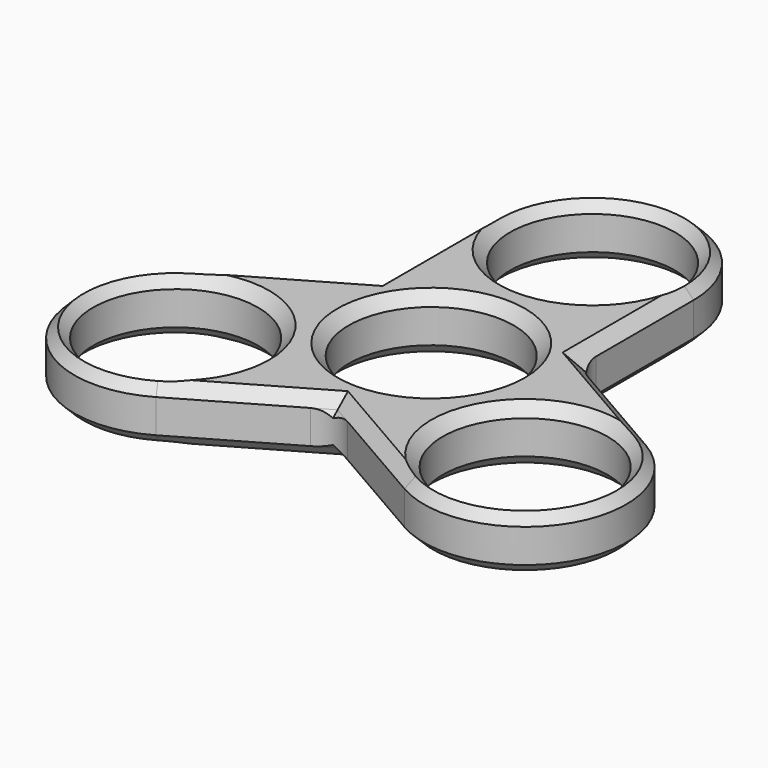
from build123d import *

# Parameters (mm, degrees)
F0_R          = 11.05
F1_DEPTH      = 7.5
F2_T4_DEPTH   = 23.0632958479
F2_T9_DEPTH   = 23.0632958479
F2_T14_DEPTH  = 23.0632958479
F2_T27_DEPTH  = 23.0632958479
F2_T32_DEPTH  = 23.0632958479
F2_T37_DEPTH  = 23.0632958479
F2_T50_DEPTH  = 23.0632958479
F2_T55_DEPTH  = 23.0632958479
F2_T60_DEPTH  = 23.0632958479
F2_T65_DEPTH  = 23.0632958479
F2_T70_DEPTH  = 23.0632958479
F2_T75_DEPTH  = 23.0632958479
F2_T78_ANGLE  = 180
F2_T80_ANGLE  = 180
F2_T82_ANGLE  = 180
F2_T84_ANGLE  = 180
F2_T86_ANGLE  = 180
F2_T88_ANGLE  = 180
F2_T93_DEPTH  = 23.0632958479
F2_T97_DEPTH  = 23.0632958479
F2_T104_DEPTH = 23.0632958479
F2_T108_DEPTH = 23.0632958479
F2_T115_DEPTH = 23.0632958479
F2_T119_DEPTH = 23.0632958479
F2_T126_DEPTH = 23.0632958479
F2_T130_DEPTH = 23.0632958479
F2_T137_DEPTH = 23.0632958479
F2_T141_DEPTH = 23.0632958479
F2_T148_DEPTH = 23.0632958479
F2_T152_DEPTH = 23.0632958479
F3_T4_DEPTH   = 18.9337567297
F3_T10_DEPTH  = 18.9337567297
F3_T16_DEPTH  = 18.9337567297
F3_T22_DEPTH  = 18.9337567297
F3_T28_DEPTH  = 18.9337567297
F3_T34_DEPTH  = 18.9337567297
F3_T40_DEPTH  = 18.9337567297
F3_T46_DEPTH  = 18.9337567297
F3_T52_DEPTH  = 18.9337567297
F3_T58_DEPTH  = 18.9337567297


# Not quite as in the source:
# - a fillet or chamfer that OpenCascade refuses, or shapes differently, is made with other operations: its cross-section is extruded or revolved along the edge and cut away or added


with BuildPart() as f1:
    # F0 (on Top) → F1 (new body)
    with BuildSketch(Plane.XY):
        with BuildLine():
            ThreePointArc((13.55, 27), (0, 40.55), (-13.55, 27))
            Line((-13.55, 27), (-13.55, 7.7942286341))
            Line((-13.55, 7.7942286341), (-30.1826859022, -1.8086570489))
            ThreePointArc((-30.1826859022, -1.8086570489), (-35.1423301235, -20.3183012702), (-16.6326859022, -25.2779454915))
            Line((-16.6326859022, -25.2779454915), (0, -15.6750598085))
            Line((0, -15.6750598085), (16.6326859022, -25.2779454915))
            ThreePointArc((16.6326859022, -25.2779454915), (35.1423301235, -20.3183012702), (30.1826859022, -1.8086570489))
            Line((30.1826859022, -1.8086570489), (13.55, 7.7942286341))
            Line((13.55, 7.7942286341), (13.55, 27))
        make_face()
        with Locations((-23.4076859022, -13.5433012702)):
            Circle(F0_R, mode=Mode.SUBTRACT)
        with Locations((23.4076859022, -13.5433012702)):
            Circle(F0_R, mode=Mode.SUBTRACT)
        Circle(F0_R, mode=Mode.SUBTRACT)
        with Locations((0, 27)):
            Circle(F0_R, mode=Mode.SUBTRACT)
    extrude(amount=F1_DEPTH)

    # F2: chamfer of 1.5 on 20 edges, made by hand


with BuildPart() as f2_tool2:
    # F2_s3 → F2_t4 (new body)
    with BuildSketch(Plane(origin=(-23.4201859022, -13.5216506351, 0), x_dir=(0, 0, 1), z_dir=(0.8660254038, 0.5, 0))):
        Polygon((6, 13.575), (7.5, 12.075), (7.5, 13.575), align=None)
    extrude(amount=F2_T4_DEPTH)

    split(bisect_by=Plane(origin=(-6.7875, -11.7562948564, 0), x_dir=(0, 0, 1), z_dir=(-0.5, -0.8660254038, 0)), keep=Keep.TOP)


with BuildPart() as f1_1:
    add(f1.part)

    # F2_t1: cut F2_tool2
    add(f2_tool2.part, mode=Mode.SUBTRACT)


with BuildPart() as f2_tool7:
    # F2_s8 → F2_t9 (new body)
    with BuildSketch(Plane.XZ.offset(-27)):
        Polygon((-13.55, 6), (-12.05, 7.5), (-13.55, 7.5), align=None)
    extrude(amount=F2_T9_DEPTH)

    split(bisect_by=Plane(origin=(-6.7625, 11.7129935862, 0), x_dir=(0, 0, 1), z_dir=(-0.5, 0.8660254038, 0)), keep=Keep.TOP)


with BuildPart() as f1_2:
    add(f1_1.part)

    # F2_t6: cut F2_tool7
    add(f2_tool7.part, mode=Mode.SUBTRACT)


with BuildPart() as f2_tool12:
    # F2_s13 → F2_t14 (new body)
    with BuildSketch(Plane(origin=(3.4467858029, -1.9900027112, 0), x_dir=(0, 0, 1), z_dir=(0.8660254038, -0.5, 0))):
        Polygon((6, 13.575), (7.5, 12.075), (7.5, 13.575), align=None)
    extrude(amount=F2_T14_DEPTH)

    split(bisect_by=Plane(origin=(6.7875, -11.7562948564, 0), x_dir=(0, 0, 1), z_dir=(0.5, -0.8660254038, 0)), keep=Keep.TOP)


with BuildPart() as f1_3:
    add(f1_2.part)

    # F2_t11: cut F2_tool12
    add(f2_tool12.part, mode=Mode.SUBTRACT)

    # F2_s16 → F2_t17 (revolve, cut)
    with BuildSketch(Plane.XZ.offset(13.5433012702)):
        Polygon((-12.3576859022, 6), (-10.8576859022, 7.5), (-12.3576859022, 7.5), align=None)
    revolve(axis=Axis((-23.4076859022, -13.5433012702, 7.5), (0, 0, 1)), mode=Mode.SUBTRACT)

    # F2_s18 → F2_t19 (revolve, cut)
    with BuildSketch(Plane.XZ):
        Polygon((11.05, 6), (12.55, 7.5), (11.05, 7.5), align=None)
    revolve(axis=Axis((0, 0, 7.5), (0, 0, 1)), mode=Mode.SUBTRACT)

    # F2_s20 → F2_t21 (revolve, cut)
    with BuildSketch(Plane.XZ.offset(-27)):
        Polygon((11.05, 6), (12.55, 7.5), (11.05, 7.5), align=None)
    revolve(axis=Axis((0, 27, 7.5), (0, 0, 1)), mode=Mode.SUBTRACT)

    # F2_s22 → F2_t23 (revolve, cut)
    with BuildSketch(Plane.XZ.offset(13.5433012702)):
        Polygon((34.4576859022, 6), (35.9576859022, 7.5), (34.4576859022, 7.5), align=None)
    revolve(axis=Axis((23.4076859022, -13.5433012702, 7.5), (0, 0, 1)), mode=Mode.SUBTRACT)


with BuildPart() as f2_tool25:
    # F2_s26 → F2_t27 (new body)
    with BuildSketch(Plane.XZ.offset(-27)):
        Polygon((-13.55, 1.5), (-12.05, 0), (-13.55, 0), align=None)
    extrude(amount=F2_T27_DEPTH)

    split(bisect_by=Plane(origin=(-6.7625, 11.7129935862, 0), x_dir=(0, 0, 1), z_dir=(-0.5, 0.8660254038, 0)), keep=Keep.TOP)


with BuildPart() as f1_4:
    add(f1_3.part)

    # F2_t24: cut F2_tool25
    add(f2_tool25.part, mode=Mode.SUBTRACT)


with BuildPart() as f2_tool30:
    # F2_s31 → F2_t32 (new body)
    with BuildSketch(Plane(origin=(-3.4467858029, -1.9900027112, 0), x_dir=(0, 0, 1), z_dir=(-0.8660254038, -0.5, 0))):
        Polygon((1.5, 13.525), (0, 12.025), (0, 13.525), align=None)
    extrude(amount=F2_T32_DEPTH)

    split(bisect_by=Plane.YZ.offset(-13.55), keep=Keep.BOTTOM)


with BuildPart() as f1_5:
    add(f1_4.part)

    # F2_t29: cut F2_tool30
    add(f2_tool30.part, mode=Mode.SUBTRACT)


with BuildPart() as f2_tool35:
    # F2_s36 → F2_t37 (new body)
    with BuildSketch(Plane(origin=(3.4467858029, -1.9900027112, 0), x_dir=(0, 0, 1), z_dir=(0.8660254038, -0.5, 0))):
        Polygon((1.5, 13.575), (0, 12.075), (0, 13.575), align=None)
    extrude(amount=F2_T37_DEPTH)

    split(bisect_by=Plane(origin=(6.7875, -11.7562948564, 0), x_dir=(0, 0, 1), z_dir=(0.5, -0.8660254038, 0)), keep=Keep.TOP)


with BuildPart() as f1_6:
    add(f1_5.part)

    # F2_t34: cut F2_tool35
    add(f2_tool35.part, mode=Mode.SUBTRACT)

    # F2_s39 → F2_t40 (revolve, cut)
    with BuildSketch(Plane.XZ.offset(13.5433012702)):
        Polygon((34.4576859022, 1.5), (35.9576859022, 0), (34.4576859022, 0), align=None)
    revolve(axis=Axis((23.4076859022, -13.5433012702, 0), (0, 0, 1)), mode=Mode.SUBTRACT)

    # F2_s41 → F2_t42 (revolve, cut)
    with BuildSketch(Plane.XZ):
        Polygon((11.05, 1.5), (12.55, 0), (11.05, 0), align=None)
    revolve(axis=Axis((0, 0, 0), (0, 0, 1)), mode=Mode.SUBTRACT)

    # F2_s43 → F2_t44 (revolve, cut)
    with BuildSketch(Plane.XZ.offset(13.5433012702)):
        Polygon((-12.3576859022, 1.5), (-10.8576859022, 0), (-12.3576859022, 0), align=None)
    revolve(axis=Axis((-23.4076859022, -13.5433012702, 0), (0, 0, 1)), mode=Mode.SUBTRACT)

    # F2_s45 → F2_t46 (revolve, cut)
    with BuildSketch(Plane.XZ.offset(-27)):
        Polygon((11.05, 1.5), (12.55, 0), (11.05, 0), align=None)
    revolve(axis=Axis((0, 27, 0), (0, 0, 1)), mode=Mode.SUBTRACT)


with BuildPart() as f2_tool48:
    # F2_s49 → F2_t50 (new body)
    with BuildSketch(Plane(origin=(-23.4201859022, -13.5216506351, 0), x_dir=(0, 0, 1), z_dir=(0.8660254038, 0.5, 0))):
        Polygon((1.5, 13.575), (0, 12.075), (0, 13.575), align=None)
    extrude(amount=F2_T50_DEPTH)

    split(bisect_by=Plane(origin=(-6.7875, -11.7562948564, 0), x_dir=(0, 0, 1), z_dir=(-0.5, -0.8660254038, 0)), keep=Keep.TOP)


with BuildPart() as f1_7:
    add(f1_6.part)

    # F2_t47: cut F2_tool48
    add(f2_tool48.part, mode=Mode.SUBTRACT)


with BuildPart() as f2_tool53:
    # F2_s54 → F2_t55 (new body)
    with BuildSketch(Plane(origin=(23.4201859022, -13.5216506351, 0), x_dir=(0, 0, 1), z_dir=(-0.8660254038, 0.5, 0))):
        Polygon((1.5, 13.525), (0, 12.025), (0, 13.525), align=None)
    extrude(amount=F2_T55_DEPTH)

    split(bisect_by=Plane.YZ.offset(13.55), keep=Keep.TOP)


with BuildPart() as f1_8:
    add(f1_7.part)

    # F2_t52: cut F2_tool53
    add(f2_tool53.part, mode=Mode.SUBTRACT)


with BuildPart() as f2_tool58:
    # F2_s59 → F2_t60 (new body)
    with BuildSketch(Plane(origin=(23.4201859022, -13.5216506351, 0), x_dir=(0, 0, 1), z_dir=(-0.8660254038, 0.5, 0))):
        Polygon((6, 13.525), (7.5, 12.025), (7.5, 13.525), align=None)
    extrude(amount=F2_T60_DEPTH)

    split(bisect_by=Plane.YZ.offset(13.55), keep=Keep.TOP)


with BuildPart() as f1_9:
    add(f1_8.part)

    # F2_t57: cut F2_tool58
    add(f2_tool58.part, mode=Mode.SUBTRACT)


with BuildPart() as f2_tool63:
    # F2_s64 → F2_t65 (new body)
    with BuildSketch(Plane.XZ.offset(-3.9367041521)):
        Polygon((13.55, 1.5), (12.05, 0), (13.55, 0), align=None)
    extrude(amount=-F2_T65_DEPTH)

    split(bisect_by=Plane(origin=(6.7625, 11.7129935862, 0), x_dir=(0, 0, 1), z_dir=(0.5, 0.8660254038, 0)), keep=Keep.TOP)


with BuildPart() as f1_10:
    add(f1_9.part)

    # F2_t62: cut F2_tool63
    add(f2_tool63.part, mode=Mode.SUBTRACT)


with BuildPart() as f2_tool68:
    # F2_s69 → F2_t70 (new body)
    with BuildSketch(Plane.XZ.offset(-3.9367041521)):
        Polygon((13.55, 6), (12.05, 7.5), (13.55, 7.5), align=None)
    extrude(amount=-F2_T70_DEPTH)

    split(bisect_by=Plane(origin=(6.7625, 11.7129935862, 0), x_dir=(0, 0, 1), z_dir=(0.5, 0.8660254038, 0)), keep=Keep.TOP)


with BuildPart() as f1_11:
    add(f1_10.part)

    # F2_t67: cut F2_tool68
    add(f2_tool68.part, mode=Mode.SUBTRACT)


with BuildPart() as f2_tool73:
    # F2_s74 → F2_t75 (new body)
    with BuildSketch(Plane(origin=(-3.4467858029, -1.9900027112, 0), x_dir=(0, 0, 1), z_dir=(-0.8660254038, -0.5, 0))):
        Polygon((6, 13.525), (7.5, 12.025), (7.5, 13.525), align=None)
    extrude(amount=F2_T75_DEPTH)

    split(bisect_by=Plane.YZ.offset(-13.55), keep=Keep.BOTTOM)


with BuildPart() as f1_12:
    add(f1_11.part)

    # F2_t72: cut F2_tool73
    add(f2_tool73.part, mode=Mode.SUBTRACT)

    # F2_s77 → F2_t78 (revolve, cut)
    with BuildSketch(Plane(origin=(-23.4201859022, -13.5216506351, 0), x_dir=(0, 0, 1), z_dir=(0.8660254038, 0.5, 0))):
        Polygon((6, -13.525), (7.5, -12.025), (7.5, -13.525), align=None)
    revolve(axis=Axis((-23.4076859022, -13.5433012702, 7.5), (0, 0, 1)), revolution_arc=F2_T78_ANGLE, mode=Mode.SUBTRACT)

    # F2_s79 → F2_t80 (revolve, cut)
    with BuildSketch(Plane.XZ.offset(-27)):
        Polygon((13.55, 6), (12.05, 7.5), (13.55, 7.5), align=None)
    revolve(axis=Axis((0, 27, 7.5), (0, 0, 1)), revolution_arc=F2_T80_ANGLE, mode=Mode.SUBTRACT)

    # F2_s81 → F2_t82 (revolve, cut)
    with BuildSketch(Plane.XZ.offset(-27)):
        Polygon((13.55, 1.5), (12.05, 0), (13.55, 0), align=None)
    revolve(axis=Axis((0, 27, 0), (0, 0, 1)), revolution_arc=F2_T82_ANGLE, mode=Mode.SUBTRACT)

    # F2_s83 → F2_t84 (revolve, cut)
    with BuildSketch(Plane(origin=(23.4201859022, -13.5216506351, 0), x_dir=(0, 0, 1), z_dir=(-0.8660254038, 0.5, 0))):
        Polygon((6, -13.575), (7.5, -12.075), (7.5, -13.575), align=None)
    revolve(axis=Axis((23.4076859022, -13.5433012702, 7.5), (0, 0, 1)), revolution_arc=F2_T84_ANGLE, mode=Mode.SUBTRACT)

    # F2_s85 → F2_t86 (revolve, cut)
    with BuildSketch(Plane(origin=(23.4201859022, -13.5216506351, 0), x_dir=(0, 0, 1), z_dir=(-0.8660254038, 0.5, 0))):
        Polygon((1.5, -13.575), (0, -12.075), (0, -13.575), align=None)
    revolve(axis=Axis((23.4076859022, -13.5433012702, 0), (0, 0, 1)), revolution_arc=F2_T86_ANGLE, mode=Mode.SUBTRACT)

    # F2_s87 → F2_t88 (revolve, cut)
    with BuildSketch(Plane(origin=(-23.4201859022, -13.5216506351, 0), x_dir=(0, 0, 1), z_dir=(0.8660254038, 0.5, 0))):
        Polygon((1.5, -13.525), (0, -12.025), (0, -13.525), align=None)
    revolve(axis=Axis((-23.4076859022, -13.5433012702, 0), (0, 0, 1)), revolution_arc=F2_T88_ANGLE, mode=Mode.SUBTRACT)


with BuildPart() as f2_tool91:
    # F2_s92 → F2_t93 (new body)
    with BuildSketch(Plane(origin=(-23.4201859022, -13.5216506351, 0), x_dir=(0, 0, 1), z_dir=(0.8660254038, 0.5, 0))):
        Polygon((6, 13.575), (7.5, 12.075), (7.5, 13.575), align=None)
    extrude(amount=F2_T93_DEPTH)

    split(bisect_by=Plane(origin=(-6.7875, -11.7562948564, 0), x_dir=(0, 0, 1), z_dir=(0.5, 0.8660254038, 0)), keep=Keep.TOP)


with BuildPart() as f2_tool95:
    # F2_s96 → F2_t97 (new body)
    with BuildSketch(Plane(origin=(3.4467858029, -1.9900027112, 0), x_dir=(0, 0, 1), z_dir=(0.8660254038, -0.5, 0))):
        Polygon((6, 13.575), (7.5, 12.075), (7.5, 13.575), align=None)
    extrude(amount=F2_T97_DEPTH)

    split(bisect_by=Plane(origin=(6.7875, -11.7562948564, 0), x_dir=(0, 0, 1), z_dir=(-0.5, 0.8660254038, 0)), keep=Keep.TOP)


with BuildPart() as f2_tool91_1:
    add(f2_tool91.part)

    # F2_t99: intersect F2_tool95
    add(f2_tool95.part, mode=Mode.INTERSECT)


with BuildPart() as f1_13:
    add(f1_12.part)

    # F2_t89: cut F2_tool91
    add(f2_tool91_1.part, mode=Mode.SUBTRACT)


with BuildPart() as f2_tool102:
    # F2_s103 → F2_t104 (new body)
    with BuildSketch(Plane.XZ.offset(-27)):
        Polygon((-13.55, 6), (-12.05, 7.5), (-13.55, 7.5), align=None)
    extrude(amount=F2_T104_DEPTH)

    split(bisect_by=Plane(origin=(-6.7625, 11.7129935862, 0), x_dir=(0, 0, 1), z_dir=(0.5, -0.8660254038, 0)), keep=Keep.TOP)


with BuildPart() as f2_tool106:
    # F2_s107 → F2_t108 (new body)
    with BuildSketch(Plane(origin=(-3.4467858029, -1.9900027112, 0), x_dir=(0, 0, 1), z_dir=(-0.8660254038, -0.5, 0))):
        Polygon((6, 13.525), (7.5, 12.025), (7.5, 13.525), align=None)
    extrude(amount=F2_T108_DEPTH)

    split(bisect_by=Plane.YZ.offset(-13.55), keep=Keep.TOP)


with BuildPart() as f2_tool102_1:
    add(f2_tool102.part)

    # F2_t110: intersect F2_tool106
    add(f2_tool106.part, mode=Mode.INTERSECT)


with BuildPart() as f1_14:
    add(f1_13.part)

    # F2_t100: cut F2_tool102
    add(f2_tool102_1.part, mode=Mode.SUBTRACT)


with BuildPart() as f2_tool113:
    # F2_s114 → F2_t115 (new body)
    with BuildSketch(Plane.XZ.offset(-27)):
        Polygon((-13.55, 1.5), (-12.05, 0), (-13.55, 0), align=None)
    extrude(amount=F2_T115_DEPTH)

    split(bisect_by=Plane(origin=(-6.7625, 11.7129935862, 0), x_dir=(0, 0, 1), z_dir=(0.5, -0.8660254038, 0)), keep=Keep.TOP)


with BuildPart() as f2_tool117:
    # F2_s118 → F2_t119 (new body)
    with BuildSketch(Plane(origin=(-3.4467858029, -1.9900027112, 0), x_dir=(0, 0, 1), z_dir=(-0.8660254038, -0.5, 0))):
        Polygon((1.5, 13.525), (0, 12.025), (0, 13.525), align=None)
    extrude(amount=F2_T119_DEPTH)

    split(bisect_by=Plane.YZ.offset(-13.55), keep=Keep.TOP)


with BuildPart() as f2_tool113_1:
    add(f2_tool113.part)

    # F2_t121: intersect F2_tool117
    add(f2_tool117.part, mode=Mode.INTERSECT)


with BuildPart() as f1_15:
    add(f1_14.part)

    # F2_t111: cut F2_tool113
    add(f2_tool113_1.part, mode=Mode.SUBTRACT)


with BuildPart() as f2_tool124:
    # F2_s125 → F2_t126 (new body)
    with BuildSketch(Plane(origin=(-23.4201859022, -13.5216506351, 0), x_dir=(0, 0, 1), z_dir=(0.8660254038, 0.5, 0))):
        Polygon((1.5, 13.575), (0, 12.075), (0, 13.575), align=None)
    extrude(amount=F2_T126_DEPTH)

    split(bisect_by=Plane(origin=(-6.7875, -11.7562948564, 0), x_dir=(0, 0, 1), z_dir=(0.5, 0.8660254038, 0)), keep=Keep.TOP)


with BuildPart() as f2_tool128:
    # F2_s129 → F2_t130 (new body)
    with BuildSketch(Plane(origin=(3.4467858029, -1.9900027112, 0), x_dir=(0, 0, 1), z_dir=(0.8660254038, -0.5, 0))):
        Polygon((1.5, 13.575), (0, 12.075), (0, 13.575), align=None)
    extrude(amount=F2_T130_DEPTH)

    split(bisect_by=Plane(origin=(6.7875, -11.7562948564, 0), x_dir=(0, 0, 1), z_dir=(-0.5, 0.8660254038, 0)), keep=Keep.TOP)


with BuildPart() as f2_tool124_1:
    add(f2_tool124.part)

    # F2_t132: intersect F2_tool128
    add(f2_tool128.part, mode=Mode.INTERSECT)


with BuildPart() as f1_16:
    add(f1_15.part)

    # F2_t122: cut F2_tool124
    add(f2_tool124_1.part, mode=Mode.SUBTRACT)


with BuildPart() as f2_tool135:
    # F2_s136 → F2_t137 (new body)
    with BuildSketch(Plane(origin=(23.4201859022, -13.5216506351, 0), x_dir=(0, 0, 1), z_dir=(-0.8660254038, 0.5, 0))):
        Polygon((1.5, 13.525), (0, 12.025), (0, 13.525), align=None)
    extrude(amount=F2_T137_DEPTH)

    split(bisect_by=Plane.YZ.offset(13.55), keep=Keep.BOTTOM)


with BuildPart() as f2_tool139:
    # F2_s140 → F2_t141 (new body)
    with BuildSketch(Plane.XZ.offset(-3.9367041521)):
        Polygon((13.55, 1.5), (12.05, 0), (13.55, 0), align=None)
    extrude(amount=-F2_T141_DEPTH)

    split(bisect_by=Plane(origin=(6.7625, 11.7129935862, 0), x_dir=(0, 0, 1), z_dir=(-0.5, -0.8660254038, 0)), keep=Keep.TOP)


with BuildPart() as f2_tool135_1:
    add(f2_tool135.part)

    # F2_t143: intersect F2_tool139
    add(f2_tool139.part, mode=Mode.INTERSECT)


with BuildPart() as f1_17:
    add(f1_16.part)

    # F2_t133: cut F2_tool135
    add(f2_tool135_1.part, mode=Mode.SUBTRACT)


with BuildPart() as f2_tool146:
    # F2_s147 → F2_t148 (new body)
    with BuildSketch(Plane(origin=(23.4201859022, -13.5216506351, 0), x_dir=(0, 0, 1), z_dir=(-0.8660254038, 0.5, 0))):
        Polygon((6, 13.525), (7.5, 12.025), (7.5, 13.525), align=None)
    extrude(amount=F2_T148_DEPTH)

    split(bisect_by=Plane.YZ.offset(13.55), keep=Keep.BOTTOM)


with BuildPart() as f2_tool150:
    # F2_s151 → F2_t152 (new body)
    with BuildSketch(Plane.XZ.offset(-3.9367041521)):
        Polygon((13.55, 6), (12.05, 7.5), (13.55, 7.5), align=None)
    extrude(amount=-F2_T152_DEPTH)

    split(bisect_by=Plane(origin=(6.7625, 11.7129935862, 0), x_dir=(0, 0, 1), z_dir=(-0.5, -0.8660254038, 0)), keep=Keep.TOP)


with BuildPart() as f2_tool146_1:
    add(f2_tool146.part)

    # F2_t154: intersect F2_tool150
    add(f2_tool150.part, mode=Mode.INTERSECT)


with BuildPart() as f1_18:
    add(f1_17.part)

    # F2_t144: cut F2_tool146
    add(f2_tool146_1.part, mode=Mode.SUBTRACT)

    # F3: fillet of radius 5 on 3 edges, made by hand


with BuildPart() as f3_tool2:
    # F3_s3 → F3_t4 (new body)
    with BuildSketch(Plane.XY.offset(-5.7168783649)):
        with BuildLine():
            ThreePointArc((-16.05, 6.3508529611), (-14.2198729811, 8.18097998), (-13.55, 10.68097998))
            Line((-13.55, 10.68097998), (-13.55, 7.7942286341))
            Line((-13.55, 7.7942286341), (-16.05, 6.3508529611))
        make_face()
    extrude(amount=F3_T4_DEPTH)

    split(bisect_by=Plane(origin=(-6.025, 0, -6.025), x_dir=(0, 1, 0), z_dir=(0.7071067812, 0, 0.7071067812)), keep=Keep.TOP)

    split(bisect_by=Plane(origin=(-4.88125, 8.4545730044, 9.7625), x_dir=(0.8660254038, 0.5, 0), z_dir=(0.3535533906, -0.6123724357, -0.7071067812)), keep=Keep.TOP)


with BuildPart() as f1_19:
    add(f1_18.part)

    # F3_t1: union F3_tool2
    add(f3_tool2.part)


with BuildPart() as f3_tool8:
    # F3_s9 → F3_t10 (new body)
    with BuildSketch(Plane.XY.offset(-5.7168783649)):
        with BuildLine():
            ThreePointArc((-16.05, 6.3508529611), (-14.2198729811, 8.18097998), (-13.55, 10.68097998))
            Line((-13.55, 10.68097998), (-13.55, 7.7942286341))
            Line((-13.55, 7.7942286341), (-16.05, 6.3508529611))
        make_face()
    extrude(amount=F3_T10_DEPTH)

    split(bisect_by=Plane(origin=(-9.775, 0, 9.775), x_dir=(0, 1, 0), z_dir=(0.7071067812, 0, -0.7071067812)), keep=Keep.TOP)

    split(bisect_by=Plane(origin=(-3.00625, 5.2069777403, -6.0125), x_dir=(0.8660254038, 0.5, 0), z_dir=(0.3535533906, -0.6123724357, 0.7071067812)), keep=Keep.TOP)


with BuildPart() as f1_20:
    add(f1_19.part)

    # F3_t7: union F3_tool8
    add(f3_tool8.part)


with BuildPart() as f3_tool14:
    # F3_s15 → F3_t16 (new body)
    with BuildSketch(Plane.XY.offset(-5.7168783649)):
        with BuildLine():
            ThreePointArc((-16.05, 6.3508529611), (-14.2198729811, 8.18097998), (-13.55, 10.68097998))
            Line((-13.55, 10.68097998), (-13.55, 7.7942286341))
            Line((-13.55, 7.7942286341), (-16.05, 6.3508529611))
        make_face()
    extrude(amount=F3_T16_DEPTH)

    split(bisect_by=Plane(origin=(-3.00625, 5.2069777403, -6.0125), x_dir=(-0.8660254038, -0.5, 0), z_dir=(-0.3535533906, 0.6123724357, -0.7071067812)), keep=Keep.TOP)

    split(bisect_by=Plane(origin=(-4.88125, 8.4545730044, 9.7625), x_dir=(-0.8660254038, -0.5, 0), z_dir=(-0.3535533906, 0.6123724357, 0.7071067812)), keep=Keep.TOP)


with BuildPart() as f1_21:
    add(f1_20.part)

    # F3_t13: union F3_tool14
    add(f3_tool14.part)


with BuildPart() as f3_tool20:
    # F3_s21 → F3_t22 (new body)
    with BuildSketch(Plane.XY.offset(-5.7168783649)):
        with BuildLine():
            ThreePointArc((-16.05, 6.3508529611), (-14.2198729811, 8.18097998), (-13.55, 10.68097998))
            Line((-13.55, 10.68097998), (-13.55, 7.7942286341))
            Line((-13.55, 7.7942286341), (-16.05, 6.3508529611))
        make_face()
    extrude(amount=F3_T22_DEPTH)

    split(bisect_by=Plane(origin=(-3.00625, 5.2069777403, -6.0125), x_dir=(0.8660254038, 0.5, 0), z_dir=(0.3535533906, -0.6123724357, 0.7071067812)), keep=Keep.TOP)

    split(bisect_by=Plane(origin=(-4.88125, 8.4545730044, 9.7625), x_dir=(0.8660254038, 0.5, 0), z_dir=(0.3535533906, -0.6123724357, -0.7071067812)), keep=Keep.TOP)


with BuildPart() as f1_22:
    add(f1_21.part)

    # F3_t19: union F3_tool20
    add(f3_tool20.part)


with BuildPart() as f3_tool26:
    # F3_s27 → F3_t28 (new body)
    with BuildSketch(Plane.XY.offset(-5.7168783649)):
        with BuildLine():
            ThreePointArc((13.55, 10.68097998), (14.2198729811, 8.18097998), (16.05, 6.3508529611))
            Line((16.05, 6.3508529611), (13.55, 7.7942286341))
            Line((13.55, 7.7942286341), (13.55, 10.68097998))
        make_face()
    extrude(amount=F3_T28_DEPTH)

    split(bisect_by=Plane(origin=(4.88125, 8.4545730044, 9.7625), x_dir=(0.8660254038, -0.5, 0), z_dir=(-0.3535533906, -0.6123724357, -0.7071067812)), keep=Keep.TOP)

    split(bisect_by=Plane(origin=(3.00625, 5.2069777403, -6.0125), x_dir=(0.8660254038, -0.5, 0), z_dir=(-0.3535533906, -0.6123724357, 0.7071067812)), keep=Keep.TOP)


with BuildPart() as f1_23:
    add(f1_22.part)

    # F3_t25: union F3_tool26
    add(f3_tool26.part)


with BuildPart() as f3_tool32:
    # F3_s33 → F3_t34 (new body)
    with BuildSketch(Plane.XY.offset(-5.7168783649)):
        with BuildLine():
            ThreePointArc((13.55, 10.68097998), (14.2198729811, 8.18097998), (16.05, 6.3508529611))
            Line((16.05, 6.3508529611), (13.55, 7.7942286341))
            Line((13.55, 7.7942286341), (13.55, 10.68097998))
        make_face()
    extrude(amount=F3_T34_DEPTH)

    split(bisect_by=Plane(origin=(9.775, 0, 9.775), x_dir=(0, 1, 0), z_dir=(-0.7071067812, 0, -0.7071067812)), keep=Keep.TOP)

    split(bisect_by=Plane(origin=(6.025, 0, -6.025), x_dir=(0, 1, 0), z_dir=(-0.7071067812, 0, 0.7071067812)), keep=Keep.TOP)


with BuildPart() as f1_24:
    add(f1_23.part)

    # F3_t31: union F3_tool32
    add(f3_tool32.part)


with BuildPart() as f3_tool38:
    # F3_s39 → F3_t40 (new body)
    with BuildSketch(Plane.XY.offset(-5.7168783649)):
        with BuildLine():
            ThreePointArc((-2.5, -17.1184354815), (0, -16.4485625004), (2.5, -17.1184354815))
            Line((2.5, -17.1184354815), (0, -15.6750598085))
            Line((0, -15.6750598085), (-2.5, -17.1184354815))
        make_face()
    extrude(amount=F3_T40_DEPTH)

    split(bisect_by=Plane(origin=(-3.01875, -5.2286283753, -6.0375), x_dir=(-0.8660254038, 0.5, 0), z_dir=(0.3535533906, 0.6123724357, 0.7071067812)), keep=Keep.TOP)

    split(bisect_by=Plane(origin=(4.89375, -8.4762236395, 9.7875), x_dir=(-0.8660254038, -0.5, 0), z_dir=(-0.3535533906, 0.6123724357, -0.7071067812)), keep=Keep.TOP)


with BuildPart() as f1_25:
    add(f1_24.part)

    # F3_t37: union F3_tool38
    add(f3_tool38.part)


with BuildPart() as f3_tool44:
    # F3_s45 → F3_t46 (new body)
    with BuildSketch(Plane.XY.offset(-5.7168783649)):
        with BuildLine():
            ThreePointArc((-2.5, -17.1184354815), (0, -16.4485625004), (2.5, -17.1184354815))
            Line((2.5, -17.1184354815), (0, -15.6750598085))
            Line((0, -15.6750598085), (-2.5, -17.1184354815))
        make_face()
    extrude(amount=F3_T46_DEPTH)

    split(bisect_by=Plane(origin=(-4.89375, -8.4762236395, 9.7875), x_dir=(-0.8660254038, 0.5, 0), z_dir=(0.3535533906, 0.6123724357, -0.7071067812)), keep=Keep.TOP)

    split(bisect_by=Plane(origin=(3.01875, -5.2286283753, -6.0375), x_dir=(-0.8660254038, -0.5, 0), z_dir=(-0.3535533906, 0.6123724357, 0.7071067812)), keep=Keep.TOP)


with BuildPart() as f1_26:
    add(f1_25.part)

    # F3_t43: union F3_tool44
    add(f3_tool44.part)


with BuildPart() as f3_tool50:
    # F3_s51 → F3_t52 (new body)
    with BuildSketch(Plane.XY.offset(-5.7168783649)):
        with BuildLine():
            ThreePointArc((-2.5, -17.1184354815), (0, -16.4485625004), (2.5, -17.1184354815))
            Line((2.5, -17.1184354815), (0, -15.6750598085))
            Line((0, -15.6750598085), (-2.5, -17.1184354815))
        make_face()
    extrude(amount=F3_T52_DEPTH)

    split(bisect_by=Plane(origin=(4.89375, -8.4762236395, 9.7875), x_dir=(0.8660254038, 0.5, 0), z_dir=(0.3535533906, -0.6123724357, 0.7071067812)), keep=Keep.TOP)

    split(bisect_by=Plane(origin=(3.01875, -5.2286283753, -6.0375), x_dir=(0.8660254038, 0.5, 0), z_dir=(0.3535533906, -0.6123724357, -0.7071067812)), keep=Keep.TOP)


with BuildPart() as f1_27:
    add(f1_26.part)

    # F3_t49: union F3_tool50
    add(f3_tool50.part)


with BuildPart() as f3_tool56:
    # F3_s57 → F3_t58 (new body)
    with BuildSketch(Plane.XY.offset(-5.7168783649)):
        with BuildLine():
            ThreePointArc((-2.5, -17.1184354815), (0, -16.4485625004), (2.5, -17.1184354815))
            Line((2.5, -17.1184354815), (0, -15.6750598085))
            Line((0, -15.6750598085), (-2.5, -17.1184354815))
        make_face()
    extrude(amount=F3_T58_DEPTH)

    split(bisect_by=Plane(origin=(4.89375, -8.4762236395, 9.7875), x_dir=(-0.8660254038, -0.5, 0), z_dir=(-0.3535533906, 0.6123724357, -0.7071067812)), keep=Keep.TOP)

    split(bisect_by=Plane(origin=(3.01875, -5.2286283753, -6.0375), x_dir=(-0.8660254038, -0.5, 0), z_dir=(-0.3535533906, 0.6123724357, 0.7071067812)), keep=Keep.TOP)


with BuildPart() as f1_28:
    add(f1_27.part)

    # F3_t55: union F3_tool56
    add(f3_tool56.part)


solid = f1_28.part
